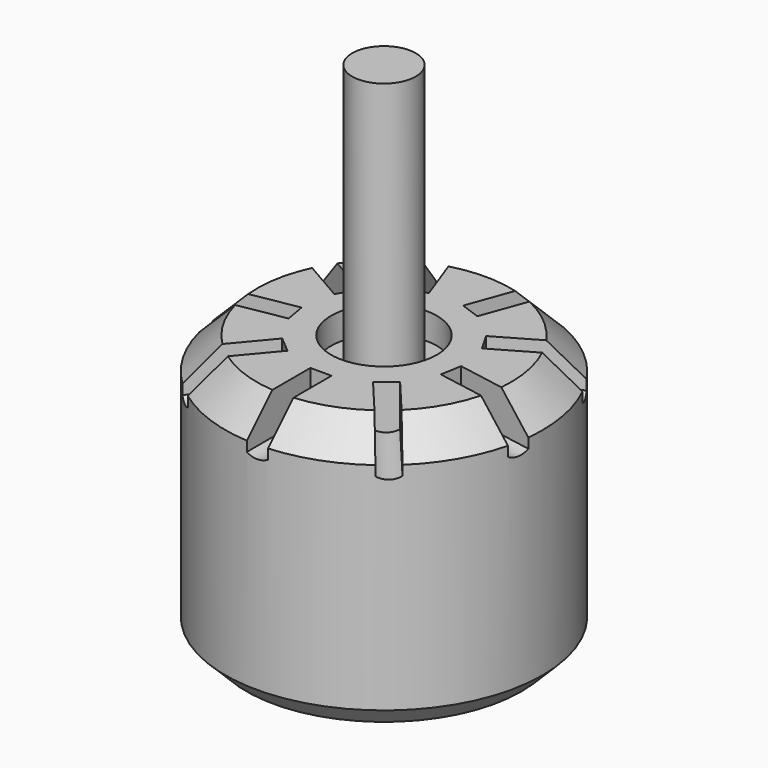
from build123d import *

# Parameters (mm, degrees)
F0_R             = 15
F1_DEPTH         = 25.4
F2_SIZE          = 3
F3_SIZE          = 2
F4_R             = 5
F5_DEPTH         = 2.5
F6_R             = 3
F7_DEPTH         = 25
F10_DEPTH        = 7.53734
F10_COPIES_COUNT = 9


# Not quite as in the source:
# - a pattern or mirror of a feature is missing from the dataset's text; its kind, count and spacing are read off the source's solid


with BuildPart() as f1:
    # F0 (on Top) → F1 (new body)
    with BuildSketch(Plane.XY):
        Circle(F0_R)
    extrude(amount=F1_DEPTH)

    # F2
    f2_edges = [f1.edges().sort_by_distance(p)[0] for p in [
        (-15, 0, 25.4),
    ]]
    chamfer(f2_edges, length=F2_SIZE)

    # F3
    f3_edges = [f1.edges().sort_by_distance(p)[0] for p in [
        (-15, 0, 0),
    ]]
    chamfer(f3_edges, length=F3_SIZE)

    # F4 (on face) → F5 (cut)
    with BuildSketch(Plane.XY.offset(25.4)):
        Circle(F4_R)
    extrude(amount=-F5_DEPTH, mode=Mode.SUBTRACT)

    # F6 (on face) → F7 (join)
    with BuildSketch(Plane.XY.offset(22.9)):
        Circle(F6_R)
    extrude(amount=F7_DEPTH)

    # F9 (on offset) → F10 (cut)
    with BuildSketch(Plane.XZ.offset(15)):
        with BuildLine():
            Line((1.0176621057, 25.4637251124), (-0.9823378943, 25.4637251124))
            Line((-0.9823378943, 25.4637251124), (-0.9823378943, 21.4637251124))
            ThreePointArc((-0.9823378943, 21.4637251124), (0.0176621057, 21.1957759199), (1.0176621057, 21.4637251124))
            Line((1.0176621057, 21.4637251124), (1.0176621057, 25.4637251124))
        make_face()
    f10 = extrude(amount=-F10_DEPTH, mode=Mode.SUBTRACT)

    # F10_copies: F10 ×9 about axis
    f10_copies_axis = Axis((0, 0, 0), (0, 0, 1))
    for i in range(1, F10_COPIES_COUNT):
        add(f10.rotate(f10_copies_axis, i * 360 / F10_COPIES_COUNT), mode=Mode.SUBTRACT)


solid = f1.part
